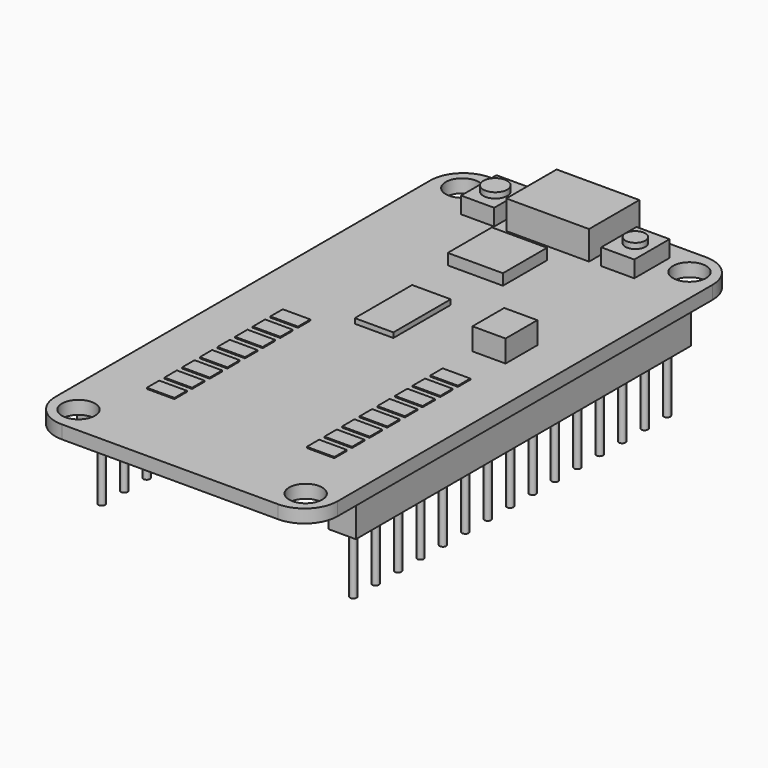
from build123d import *

# Parameters (mm, degrees)
F0_R      = 1.5
F1_DEPTH  = 1.2
F2_W      = 2.5
F2_H      = 38
F3_DEPTH  = 2.8
F4_R      = 0.3
F5_DEPTH  = 5.5
F7_W      = 3
F7_H      = 4
F8_DEPTH  = 1.5
F9_R      = 1.0863187535
F10_DEPTH = 0.5
F9_R_2    = 0.9
F11_W     = 2.5
F11_H     = 1.4
F12_DEPTH = 0.1
F6_W      = 7.5
F6_H      = 5.7
F13_DEPTH = 2.6
F14_W     = 3
F14_H     = 3.6
F15_DEPTH = 2
F16_W     = 3.5
F16_H     = 6.5
F17_DEPTH = 1.65
F18_W     = 5
F18_H     = 5
F19_DEPTH = 1


# Not quite as in the source:
# - a feature names something its author has since deleted; it is built from what else it names


with BuildPart() as f1:
    # F0 (on Top) → F1 (new body)
    with BuildSketch(Plane.XY):
        with BuildLine():
            Line((9.8, 24.25), (-9.8, 24.25))
            ThreePointArc((-9.8, 24.25), (-11.9213203436, 23.3713203436), (-12.8, 21.25))
            Line((-12.8, 21.25), (-12.8, -21.25))
            ThreePointArc((-12.8, -21.25), (-11.9213203436, -23.3713203436), (-9.8, -24.25))
            Line((-9.8, -24.25), (9.8, -24.25))
            ThreePointArc((9.8, -24.25), (11.9213203436, -23.3713203436), (12.8, -21.25))
            Line((12.8, -21.25), (12.8, 21.25))
            ThreePointArc((12.8, 21.25), (11.9213203436, 23.3713203436), (9.8, 24.25))
        make_face()
        with Locations((-10.3, -21.75)):
            Circle(F0_R, mode=Mode.SUBTRACT)
        with Locations((10.3, -21.75)):
            Circle(F0_R, mode=Mode.SUBTRACT)
        with Locations((-10.3, 21.75)):
            Circle(F0_R, mode=Mode.SUBTRACT)
        with Locations((10.3, 21.75)):
            Circle(F0_R, mode=Mode.SUBTRACT)
    extrude(amount=F1_DEPTH)

    # F16 (on Top) → F17 (join)
    with BuildSketch(Plane.XY):
        with Locations((-1.5, 4)):
            Rectangle(F16_W, F16_H)
    extrude(amount=F17_DEPTH)

    # F18 (on face) → F19 (join)
    with BuildSketch(Plane.XY.offset(1.2)):
        with Locations((-1.2, 14.35)):
            Rectangle(F18_W, F18_H)
    extrude(amount=F19_DEPTH)


with BuildPart() as f3:
    # F2 (on face) → F3 (new body)
    with BuildSketch(Plane(origin=(0, 0, 0), x_dir=(1, 0, 0), z_dir=(0, 0, -1))):
        with Locations((11.4, 0)):
            Rectangle(F2_W, F2_H)
    extrude(amount=F3_DEPTH)


with BuildPart() as f3b:
    # F2 (on face) → F3, piece 2 (new body)
    with BuildSketch(Plane(origin=(0, 0, 0), x_dir=(1, 0, 0), z_dir=(0, 0, -1))):
        with Locations((-11.4, 0)):
            Rectangle(F2_W, F2_H)
    extrude(amount=F3_DEPTH)


with BuildPart() as f5:
    # F4 (on face) → F5 (new body)
    with BuildSketch(Plane(origin=(0, 0, -2.8), x_dir=(1, 0, 0), z_dir=(0, 0, -1))):
        with Locations((-11.4, 17.7333333333)):
            Circle(F4_R)
    extrude(amount=F5_DEPTH)


with BuildPart() as f5b:
    # F4 (on face) → F5, piece 2 (new body)
    with BuildSketch(Plane(origin=(0, 0, -2.8), x_dir=(1, 0, 0), z_dir=(0, 0, -1))):
        with Locations((-11.4, 15.1933333333)):
            Circle(F4_R)
    extrude(amount=F5_DEPTH)


with BuildPart() as f5c:
    # F4 (on face) → F5, piece 3 (new body)
    with BuildSketch(Plane(origin=(0, 0, -2.8), x_dir=(1, 0, 0), z_dir=(0, 0, -1))):
        with Locations((-11.4, 12.6533333333)):
            Circle(F4_R)
    extrude(amount=F5_DEPTH)


with BuildPart() as f5d:
    # F4 (on face) → F5, piece 4 (new body)
    with BuildSketch(Plane(origin=(0, 0, -2.8), x_dir=(1, 0, 0), z_dir=(0, 0, -1))):
        with Locations((-11.4, 10.1133333333)):
            Circle(F4_R)
    extrude(amount=F5_DEPTH)


with BuildPart() as f5e:
    # F4 (on face) → F5, piece 5 (new body)
    with BuildSketch(Plane(origin=(0, 0, -2.8), x_dir=(1, 0, 0), z_dir=(0, 0, -1))):
        with Locations((-11.4, 7.5733333333)):
            Circle(F4_R)
    extrude(amount=F5_DEPTH)


with BuildPart() as f5f:
    # F4 (on face) → F5, piece 6 (new body)
    with BuildSketch(Plane(origin=(0, 0, -2.8), x_dir=(1, 0, 0), z_dir=(0, 0, -1))):
        with Locations((-11.4, 5.0333333333)):
            Circle(F4_R)
    extrude(amount=F5_DEPTH)


with BuildPart() as f5g:
    # F4 (on face) → F5, piece 7 (new body)
    with BuildSketch(Plane(origin=(0, 0, -2.8), x_dir=(1, 0, 0), z_dir=(0, 0, -1))):
        with Locations((11.4, 17.7333333333)):
            Circle(F4_R)
    extrude(amount=F5_DEPTH)


with BuildPart() as f5h:
    # F4 (on face) → F5, piece 8 (new body)
    with BuildSketch(Plane(origin=(0, 0, -2.8), x_dir=(1, 0, 0), z_dir=(0, 0, -1))):
        with Locations((11.4, 15.1933333333)):
            Circle(F4_R)
    extrude(amount=F5_DEPTH)


with BuildPart() as f5i:
    # F4 (on face) → F5, piece 9 (new body)
    with BuildSketch(Plane(origin=(0, 0, -2.8), x_dir=(1, 0, 0), z_dir=(0, 0, -1))):
        with Locations((11.4, 12.6533333333)):
            Circle(F4_R)
    extrude(amount=F5_DEPTH)


with BuildPart() as f5j:
    # F4 (on face) → F5, piece 10 (new body)
    with BuildSketch(Plane(origin=(0, 0, -2.8), x_dir=(1, 0, 0), z_dir=(0, 0, -1))):
        with Locations((11.4, 10.1133333333)):
            Circle(F4_R)
    extrude(amount=F5_DEPTH)


with BuildPart() as f5k:
    # F4 (on face) → F5, piece 11 (new body)
    with BuildSketch(Plane(origin=(0, 0, -2.8), x_dir=(1, 0, 0), z_dir=(0, 0, -1))):
        with Locations((11.4, 7.5733333333)):
            Circle(F4_R)
    extrude(amount=F5_DEPTH)


with BuildPart() as f5l:
    # F4 (on face) → F5, piece 12 (new body)
    with BuildSketch(Plane(origin=(0, 0, -2.8), x_dir=(1, 0, 0), z_dir=(0, 0, -1))):
        with Locations((11.4, 5.0333333333)):
            Circle(F4_R)
    extrude(amount=F5_DEPTH)


with BuildPart() as f5m:
    # F4 (on face) → F5, piece 13 (new body)
    with BuildSketch(Plane(origin=(0, 0, -2.8), x_dir=(1, 0, 0), z_dir=(0, 0, -1))):
        with Locations((11.4, 2.4933333333)):
            Circle(F4_R)
    extrude(amount=F5_DEPTH)


with BuildPart() as f5n:
    # F4 (on face) → F5, piece 14 (new body)
    with BuildSketch(Plane(origin=(0, 0, -2.8), x_dir=(1, 0, 0), z_dir=(0, 0, -1))):
        with Locations((11.4, -0.0466666667)):
            Circle(F4_R)
    extrude(amount=F5_DEPTH)


with BuildPart() as f5o:
    # F4 (on face) → F5, piece 15 (new body)
    with BuildSketch(Plane(origin=(0, 0, -2.8), x_dir=(1, 0, 0), z_dir=(0, 0, -1))):
        with Locations((-11.4, 2.4933333333)):
            Circle(F4_R)
    extrude(amount=F5_DEPTH)


with BuildPart() as f5p:
    # F4 (on face) → F5, piece 16 (new body)
    with BuildSketch(Plane(origin=(0, 0, -2.8), x_dir=(1, 0, 0), z_dir=(0, 0, -1))):
        with Locations((-11.4, -0.0466666667)):
            Circle(F4_R)
    extrude(amount=F5_DEPTH)


with BuildPart() as f5q:
    # F4 (on face) → F5, piece 17 (new body)
    with BuildSketch(Plane(origin=(0, 0, -2.8), x_dir=(1, 0, 0), z_dir=(0, 0, -1))):
        with Locations((-11.4, -2.5866666667)):
            Circle(F4_R)
    extrude(amount=F5_DEPTH)


with BuildPart() as f5r:
    # F4 (on face) → F5, piece 18 (new body)
    with BuildSketch(Plane(origin=(0, 0, -2.8), x_dir=(1, 0, 0), z_dir=(0, 0, -1))):
        with Locations((-11.4, -5.1266666667)):
            Circle(F4_R)
    extrude(amount=F5_DEPTH)


with BuildPart() as f5s:
    # F4 (on face) → F5, piece 19 (new body)
    with BuildSketch(Plane(origin=(0, 0, -2.8), x_dir=(1, 0, 0), z_dir=(0, 0, -1))):
        with Locations((-11.4, -7.6666666667)):
            Circle(F4_R)
    extrude(amount=F5_DEPTH)


with BuildPart() as f5t:
    # F4 (on face) → F5, piece 20 (new body)
    with BuildSketch(Plane(origin=(0, 0, -2.8), x_dir=(1, 0, 0), z_dir=(0, 0, -1))):
        with Locations((-11.4, -10.2066666667)):
            Circle(F4_R)
    extrude(amount=F5_DEPTH)


with BuildPart() as f5u:
    # F4 (on face) → F5, piece 21 (new body)
    with BuildSketch(Plane(origin=(0, 0, -2.8), x_dir=(1, 0, 0), z_dir=(0, 0, -1))):
        with Locations((-11.4, -12.7466666667)):
            Circle(F4_R)
    extrude(amount=F5_DEPTH)


with BuildPart() as f5v:
    # F4 (on face) → F5, piece 22 (new body)
    with BuildSketch(Plane(origin=(0, 0, -2.8), x_dir=(1, 0, 0), z_dir=(0, 0, -1))):
        with Locations((11.4, -2.5866666667)):
            Circle(F4_R)
    extrude(amount=F5_DEPTH)


with BuildPart() as f5w:
    # F4 (on face) → F5, piece 23 (new body)
    with BuildSketch(Plane(origin=(0, 0, -2.8), x_dir=(1, 0, 0), z_dir=(0, 0, -1))):
        with Locations((11.4, -5.1266666667)):
            Circle(F4_R)
    extrude(amount=F5_DEPTH)


with BuildPart() as f5x:
    # F4 (on face) → F5, piece 24 (new body)
    with BuildSketch(Plane(origin=(0, 0, -2.8), x_dir=(1, 0, 0), z_dir=(0, 0, -1))):
        with Locations((11.4, -7.6666666667)):
            Circle(F4_R)
    extrude(amount=F5_DEPTH)


with BuildPart() as f5y:
    # F4 (on face) → F5, piece 25 (new body)
    with BuildSketch(Plane(origin=(0, 0, -2.8), x_dir=(1, 0, 0), z_dir=(0, 0, -1))):
        with Locations((11.4, -10.2066666667)):
            Circle(F4_R)
    extrude(amount=F5_DEPTH)


with BuildPart() as f5z:
    # F4 (on face) → F5, piece 26 (new body)
    with BuildSketch(Plane(origin=(0, 0, -2.8), x_dir=(1, 0, 0), z_dir=(0, 0, -1))):
        with Locations((11.4, -12.7466666667)):
            Circle(F4_R)
    extrude(amount=F5_DEPTH)


with BuildPart() as f5ba:
    # F4 (on face) → F5, piece 27 (new body)
    with BuildSketch(Plane(origin=(0, 0, -2.8), x_dir=(1, 0, 0), z_dir=(0, 0, -1))):
        with Locations((11.4, -15.2866666667)):
            Circle(F4_R)
    extrude(amount=F5_DEPTH)


with BuildPart() as f5bb:
    # F4 (on face) → F5, piece 28 (new body)
    with BuildSketch(Plane(origin=(0, 0, -2.8), x_dir=(1, 0, 0), z_dir=(0, 0, -1))):
        with Locations((11.4, -17.8266666667)):
            Circle(F4_R)
    extrude(amount=F5_DEPTH)


with BuildPart() as f5bc:
    # F4 (on face) → F5, piece 29 (new body)
    with BuildSketch(Plane(origin=(0, 0, -2.8), x_dir=(1, 0, 0), z_dir=(0, 0, -1))):
        with Locations((-11.4, -17.8266666667)):
            Circle(F4_R)
    extrude(amount=F5_DEPTH)


with BuildPart() as f5bd:
    # F4 (on face) → F5, piece 30 (new body)
    with BuildSketch(Plane(origin=(0, 0, -2.8), x_dir=(1, 0, 0), z_dir=(0, 0, -1))):
        with Locations((-11.4, -15.2866666667)):
            Circle(F4_R)
    extrude(amount=F5_DEPTH)


with BuildPart() as f8:
    # F7 (on face) → F8 (new body)
    with BuildSketch(Plane.XY.offset(1.2)):
        with Locations((-6.35, 20.55)):
            Rectangle(F7_W, F7_H)
    extrude(amount=F8_DEPTH)


with BuildPart() as f8b:
    # F7 (on face) → F8, piece 2 (new body)
    with BuildSketch(Plane.XY.offset(1.2)):
        with Locations((6.35, 20.55)):
            Rectangle(F7_W, F7_H)
    extrude(amount=F8_DEPTH)


with BuildPart() as f10:
    # F9 (on face) → F10 (new body)
    with BuildSketch(Plane.XY.offset(2.7)):
        with Locations((-6.35, 20.55)):
            Circle(F9_R)
    extrude(amount=F10_DEPTH)


with BuildPart() as f10b:
    # F9 (on face) → F10, piece 2 (new body)
    with BuildSketch(Plane.XY.offset(2.7)):
        with Locations((6.35, 20.55)):
            Circle(F9_R_2)
    extrude(amount=F10_DEPTH)


with BuildPart() as f12:
    # F11 (on face) → F12 (new body)
    with BuildSketch(Plane.XY.offset(1.2)):
        with Locations((-7.25, -15.55)):
            Rectangle(F11_W, F11_H)
    extrude(amount=F12_DEPTH)


with BuildPart() as f12b:
    # F11 (on face) → F12, piece 2 (new body)
    with BuildSketch(Plane.XY.offset(1.2)):
        with Locations((-7.25, -13.55)):
            Rectangle(F11_W, F11_H)
    extrude(amount=F12_DEPTH)


with BuildPart() as f12c:
    # F11 (on face) → F12, piece 3 (new body)
    with BuildSketch(Plane.XY.offset(1.2)):
        with Locations((-7.25, -11.55)):
            Rectangle(F11_W, F11_H)
    extrude(amount=F12_DEPTH)


with BuildPart() as f12d:
    # F11 (on face) → F12, piece 4 (new body)
    with BuildSketch(Plane.XY.offset(1.2)):
        with Locations((-7.25, -9.55)):
            Rectangle(F11_W, F11_H)
    extrude(amount=F12_DEPTH)


with BuildPart() as f12e:
    # F11 (on face) → F12, piece 5 (new body)
    with BuildSketch(Plane.XY.offset(1.2)):
        with Locations((-7.25, -7.55)):
            Rectangle(F11_W, F11_H)
    extrude(amount=F12_DEPTH)


with BuildPart() as f12f:
    # F11 (on face) → F12, piece 6 (new body)
    with BuildSketch(Plane.XY.offset(1.2)):
        with Locations((-7.25, -5.55)):
            Rectangle(F11_W, F11_H)
    extrude(amount=F12_DEPTH)


with BuildPart() as f12g:
    # F11 (on face) → F12, piece 7 (new body)
    with BuildSketch(Plane.XY.offset(1.2)):
        with Locations((-7.25, -3.55)):
            Rectangle(F11_W, F11_H)
    extrude(amount=F12_DEPTH)


with BuildPart() as f12h:
    # F11 (on face) → F12, piece 8 (new body)
    with BuildSketch(Plane.XY.offset(1.2)):
        with Locations((-7.25, -1.55)):
            Rectangle(F11_W, F11_H)
    extrude(amount=F12_DEPTH)


with BuildPart() as f12i:
    # F11 (on face) → F12, piece 9 (new body)
    with BuildSketch(Plane.XY.offset(1.2)):
        with Locations((7.25, -15.55)):
            Rectangle(F11_W, F11_H)
    extrude(amount=F12_DEPTH)


with BuildPart() as f12j:
    # F11 (on face) → F12, piece 10 (new body)
    with BuildSketch(Plane.XY.offset(1.2)):
        with Locations((7.25, -13.55)):
            Rectangle(F11_W, F11_H)
    extrude(amount=F12_DEPTH)


with BuildPart() as f12k:
    # F11 (on face) → F12, piece 11 (new body)
    with BuildSketch(Plane.XY.offset(1.2)):
        with Locations((7.25, -11.55)):
            Rectangle(F11_W, F11_H)
    extrude(amount=F12_DEPTH)


with BuildPart() as f12l:
    # F11 (on face) → F12, piece 12 (new body)
    with BuildSketch(Plane.XY.offset(1.2)):
        with Locations((7.25, -9.55)):
            Rectangle(F11_W, F11_H)
    extrude(amount=F12_DEPTH)


with BuildPart() as f12m:
    # F11 (on face) → F12, piece 13 (new body)
    with BuildSketch(Plane.XY.offset(1.2)):
        with Locations((7.25, -7.55)):
            Rectangle(F11_W, F11_H)
    extrude(amount=F12_DEPTH)


with BuildPart() as f12n:
    # F11 (on face) → F12, piece 14 (new body)
    with BuildSketch(Plane.XY.offset(1.2)):
        with Locations((7.25, -5.55)):
            Rectangle(F11_W, F11_H)
    extrude(amount=F12_DEPTH)


with BuildPart() as f12o:
    # F11 (on face) → F12, piece 15 (new body)
    with BuildSketch(Plane.XY.offset(1.2)):
        with Locations((7.25, -3.55)):
            Rectangle(F11_W, F11_H)
    extrude(amount=F12_DEPTH)


with BuildPart() as f12p:
    # F11 (on face) → F12, piece 16 (new body)
    with BuildSketch(Plane.XY.offset(1.2)):
        with Locations((7.25, -1.55)):
            Rectangle(F11_W, F11_H)
    extrude(amount=F12_DEPTH)


with BuildPart() as f13:
    # F6 (on face) → F13 (new body)
    with BuildSketch(Plane.XY.offset(1.2)):
        with Locations((0, 21.4)):
            Rectangle(F6_W, F6_H)
    extrude(amount=F13_DEPTH)


with BuildPart() as f15:
    # F14 (on face) → F15 (new body)
    with BuildSketch(Plane.XY.offset(1.2)):
        with Locations((7.4, 4.45)):
            Rectangle(F14_W, F14_H)
    extrude(amount=F15_DEPTH)


solid = Compound([f1.part, f3.part, f3b.part, f5.part, f5b.part, f5c.part, f5d.part, f5e.part, f5f.part, f5g.part, f5h.part, f5i.part, f5j.part, f5k.part, f5l.part, f5m.part, f5n.part, f5o.part, f5p.part, f5q.part, f5r.part, f5s.part, f5t.part, f5u.part, f5v.part, f5w.part, f5x.part, f5y.part, f5z.part, f5ba.part, f5bb.part, f5bc.part, f5bd.part, f8.part, f8b.part, f10.part, f10b.part, f12.part, f12b.part, f12c.part, f12d.part, f12e.part, f12f.part, f12g.part, f12h.part, f12i.part, f12j.part, f12k.part, f12l.part, f12m.part, f12n.part, f12o.part, f12p.part, f13.part, f15.part])
